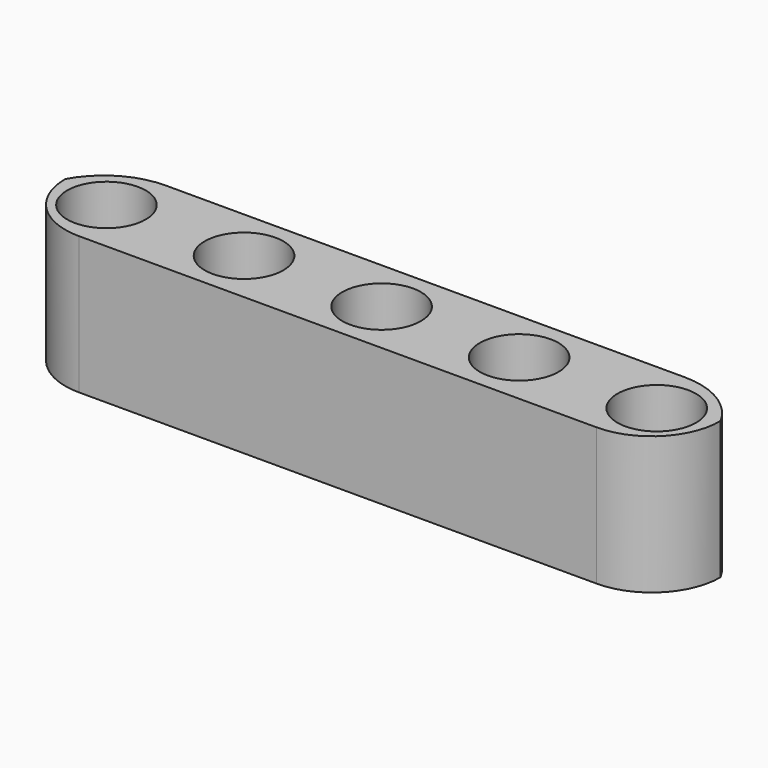
from build123d import *

# Parameters (mm, degrees)
F0_R        = 2.286
F1_DEPTH    = 8
F2_R        = 4
F3_R        = 4
F4_T1_DEPTH = 27.7658164516
F5_T1_DEPTH = 27.7658164516


# Not quite as in the source:
# - a fillet or chamfer that OpenCascade refuses, or shapes differently, is made with other operations: its cross-section is extruded or revolved along the edge and cut away or added


with BuildPart() as f1:
    # F0 (on Top) → F1 (new body)
    with BuildSketch(Plane.XY):
        Polygon((19.2099873261, 3.0477390712), (-18.8900126739, 3.0477390712), (-18.8900126739, -3.3271788533), (-17.4405010572, -3.3022609288), (19.2099873261, -3.3022609288), align=None)
        with Locations((-15.8400126739, -0.1272609288)):
            Circle(F0_R, mode=Mode.SUBTRACT)
        with Locations((-7.8400126739, -0.1272609288)):
            Circle(F0_R, mode=Mode.SUBTRACT)
        with Locations((0.1599873261, -0.1272609288)):
            Circle(F0_R, mode=Mode.SUBTRACT)
        with Locations((8.1599873261, -0.1272609288)):
            Circle(F0_R, mode=Mode.SUBTRACT)
        with Locations((16.1599873261, -0.1272609288)):
            Circle(F0_R, mode=Mode.SUBTRACT)
    extrude(amount=F1_DEPTH)

    # F2
    f2_edges = [f1.edges().sort_by_distance(p)[0] for p in [
        (-18.890013, -3.327179, 4),
    ]]
    fillet(f2_edges, radius=F2_R)

    # F3
    f3_edges = [f1.edges().sort_by_distance(p)[0] for p in [
        (19.209987, -3.302261, 4),
    ]]
    fillet(f3_edges, radius=F3_R)

    # F4: fillet of radius 4.5 on 1 edges, made by hand

    # F4_s2 → F4_t1 (cut)
    with BuildSketch(Plane.XY.offset(-9.8829082258)):
        with BuildLine():
            ThreePointArc((19.2099873261, 0.6977390712), (17.5562804933, 2.4158781586), (15.2568240358, 3.0477390712))
            Line((15.2568240358, 3.0477390712), (19.2099873261, 3.0477390712))
            Line((19.2099873261, 3.0477390712), (19.2099873261, 0.6977390712))
        make_face()
    extrude(amount=F4_T1_DEPTH, mode=Mode.SUBTRACT)

    # F5: fillet of radius 4.5 on 1 edges, made by hand

    # F5_s2 → F5_t1 (cut)
    with BuildSketch(Plane.XY.offset(-9.8829082258)):
        with BuildLine():
            ThreePointArc((-18.8900126739, 0.6977390712), (-17.2363058411, 2.4158781586), (-14.9368493836, 3.0477390712))
            Line((-14.9368493836, 3.0477390712), (-18.8900126739, 3.0477390712))
            Line((-18.8900126739, 3.0477390712), (-18.8900126739, 0.6977390712))
        make_face()
    extrude(amount=F5_T1_DEPTH, mode=Mode.SUBTRACT)


solid = f1.part
